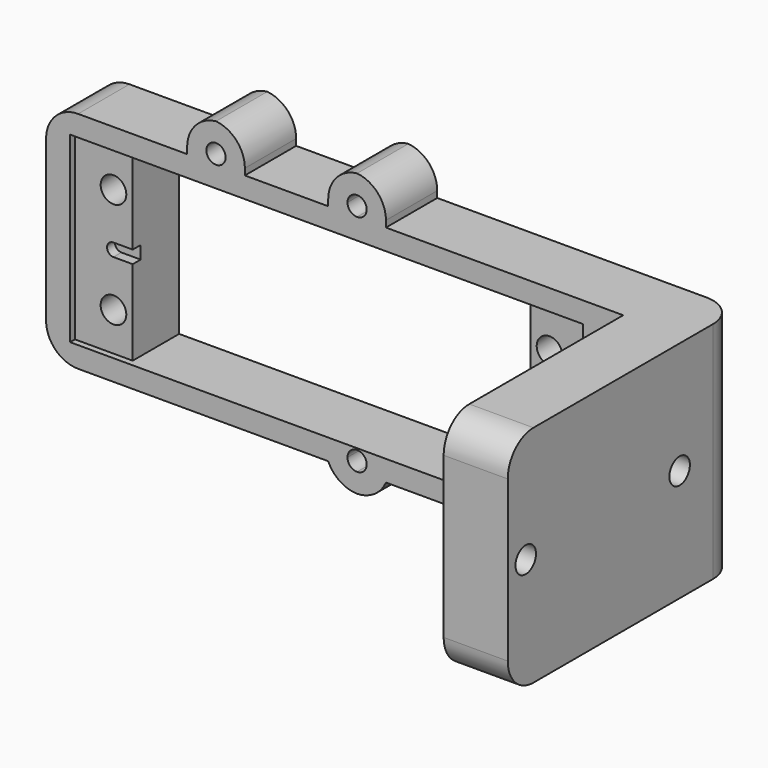
from build123d import *

# Parameters (mm, degrees)
F2_DEPTH     = 35
F4_DEPTH     = 10
F3_R         = 2
F5_DEPTH     = 0.95
F6_DEPTH     = 2.5
F7_DEPTH     = 6
F8_W         = 9
F8_H         = 9.25
F8_R         = 1.5
F8_H_2       = 6.25
F9_DEPTH     = 10
F10_DEPTH    = 10
F11_R        = 2
F12_DEPTH    = 6
F13_T1_DEPTH = 35
F13_T3_DEPTH = 35
F13_T5_DEPTH = 60
F13_T7_DEPTH = 32.9128784748


# Not quite as in the source:
# - a fillet or chamfer that OpenCascade refuses, or shapes differently, is made with other operations: its cross-section is extruded or revolved along the edge and cut away or added


with BuildPart() as f2:
    # F1 (on Top) → F2 (new body)
    with BuildSketch(Plane.XY):
        Polygon((50, -22.5), (50, 22.5), (-50, 22.5), (-50, 12.5), (40, 12.5), (40, -22.5), align=None)
    extrude(amount=F2_DEPTH)

    # F3 (on face) → F4 (cut, through all)
    with BuildSketch(Plane.XZ.offset(-12.5)):
        with BuildLine():
            Line((-37.25, 3.25), (24.75, 3.25))
            Line((24.75, 3.25), (24.75, 16.5))
            ThreePointArc((24.75, 16.5), (23.75, 17.5), (24.75, 18.5))
            Line((24.75, 18.5), (24.75, 31.75))
            Line((24.75, 31.75), (-37.25, 31.75))
            Line((-37.25, 31.75), (-37.25, 18.5))
            ThreePointArc((-37.25, 18.5), (-36.25, 17.5), (-37.25, 16.5))
            Line((-37.25, 16.5), (-37.25, 3.25))
        make_face()
        with BuildLine():
            Line((-37.25, 17.5), (-37.25, 16.5))
            ThreePointArc((-37.25, 16.5), (-36.25, 17.5), (-37.25, 18.5))
            Line((-37.25, 18.5), (-37.25, 17.5))
        make_face()
        with BuildLine():
            ThreePointArc((24.75, 18.5), (23.75, 17.5), (24.75, 16.5))
            Line((24.75, 16.5), (24.75, 17.5))
            Line((24.75, 17.5), (24.75, 18.5))
        make_face()
    extrude(amount=-F4_DEPTH, mode=Mode.SUBTRACT)

    # F3 (on face) → F5 (cut)
    with BuildSketch(Plane.XZ.offset(-12.5)):
        with BuildLine():
            Line((-43.25, 3.25), (-37.25, 3.25))
            Line((-37.25, 3.25), (-37.25, 16.5))
            Line((-37.25, 16.5), (-40.25, 16.5))
            ThreePointArc((-40.25, 16.5), (-41.25, 17.5), (-40.25, 18.5))
            Line((-40.25, 18.5), (-37.25, 18.5))
            Line((-37.25, 18.5), (-37.25, 31.75))
            Line((-37.25, 31.75), (-43.25, 31.75))
            Line((-43.25, 31.75), (-46.25, 31.75))
            Line((-46.25, 31.75), (-46.25, 3.25))
            Line((-46.25, 3.25), (-43.25, 3.25))
        make_face()
        with Locations((-40.25, 9.25)):
            Circle(F3_R, mode=Mode.SUBTRACT)
        with Locations((-40.25, 25.75)):
            Circle(F3_R, mode=Mode.SUBTRACT)
        with BuildLine():
            Line((27.75, 3.25), (30.75, 3.25))
            Line((30.75, 3.25), (33.75, 3.25))
            Line((33.75, 3.25), (33.75, 31.75))
            Line((33.75, 31.75), (30.75, 31.75))
            Line((30.75, 31.75), (24.75, 31.75))
            Line((24.75, 31.75), (24.75, 18.5))
            Line((24.75, 18.5), (27.75, 18.5))
            ThreePointArc((27.75, 18.5), (28.75, 17.5), (27.75, 16.5))
            Line((27.75, 16.5), (24.75, 16.5))
            Line((24.75, 16.5), (24.75, 3.25))
            Line((24.75, 3.25), (27.75, 3.25))
        make_face()
        with Locations((27.75, 9.25)):
            Circle(F3_R, mode=Mode.SUBTRACT)
        with Locations((27.75, 25.75)):
            Circle(F3_R, mode=Mode.SUBTRACT)
        with BuildLine():
            Line((-40.25, 16.5), (-37.25, 16.5))
            Line((-37.25, 16.5), (-37.25, 17.5))
            Line((-37.25, 17.5), (-37.25, 18.5))
            Line((-37.25, 18.5), (-40.25, 18.5))
            ThreePointArc((-40.25, 18.5), (-41.25, 17.5), (-40.25, 16.5))
        make_face()
        with BuildLine():
            Line((24.75, 17.5), (24.75, 16.5))
            Line((24.75, 16.5), (27.75, 16.5))
            ThreePointArc((27.75, 16.5), (28.75, 17.5), (27.75, 18.5))
            Line((27.75, 18.5), (24.75, 18.5))
            Line((24.75, 18.5), (24.75, 17.5))
        make_face()
    extrude(amount=-F5_DEPTH, mode=Mode.SUBTRACT)

    # F3 (on face) → F6 (cut)
    with BuildSketch(Plane.XZ.offset(-12.5)):
        with BuildLine():
            Line((-40.25, 16.5), (-37.25, 16.5))
            Line((-37.25, 16.5), (-37.25, 17.5))
            Line((-37.25, 17.5), (-37.25, 18.5))
            Line((-37.25, 18.5), (-40.25, 18.5))
            ThreePointArc((-40.25, 18.5), (-41.25, 17.5), (-40.25, 16.5))
        make_face()
        with BuildLine():
            Line((24.75, 17.5), (24.75, 16.5))
            Line((24.75, 16.5), (27.75, 16.5))
            ThreePointArc((27.75, 16.5), (28.75, 17.5), (27.75, 18.5))
            Line((27.75, 18.5), (24.75, 18.5))
            Line((24.75, 18.5), (24.75, 17.5))
        make_face()
    extrude(amount=-F6_DEPTH, mode=Mode.SUBTRACT)

    # F3 (on face) → F7 (cut)
    with BuildSketch(Plane.XZ.offset(-12.5)):
        with Locations((-40.25, 25.75)):
            Circle(F3_R)
        with Locations((-40.25, 9.25)):
            Circle(F3_R)
        with Locations((27.75, 9.25)):
            Circle(F3_R)
        with Locations((27.75, 25.75)):
            Circle(F3_R)
    extrude(amount=-F7_DEPTH, mode=Mode.SUBTRACT)

    # F8 (on face) → F9 (join, through all)
    with BuildSketch(Plane(origin=(0, 22.5, 0), x_dir=(-1, 0, 0), z_dir=(0, 1, 0))):
        with Locations((1.5, 36.375)):
            Rectangle(F8_W, F8_H)
        with Locations((1.5, 36.5)):
            Circle(F8_R, mode=Mode.SUBTRACT)
        with Locations((1.5, 0.125)):
            Rectangle(F8_W, F8_H_2)
        with Locations((1.5, 1.5)):
            Circle(F8_R, mode=Mode.SUBTRACT)
        with Locations((23.5, 36.375)):
            Rectangle(F8_W, F8_H)
        with Locations((23.5, 36.5)):
            Circle(F8_R, mode=Mode.SUBTRACT)
        with BuildLine():
            ThreePointArc((3, 36.5), (0.4393398187, 37.5606601622), (1.5000000271, 35))
            ThreePointArc((1.5000000271, 35), (2.5606601813, 35.4393398378), (3, 36.5))
        make_face()
    extrude(amount=-F9_DEPTH)

    # F8 (on face) → F10 (cut, through all)
    with BuildSketch(Plane(origin=(0, 22.5, 0), x_dir=(-1, 0, 0), z_dir=(0, 1, 0))):
        with BuildLine():
            ThreePointArc((3, 1.5), (0.4393398305, 2.560660174), (1.4999999936, 0))
            ThreePointArc((1.4999999936, 0), (2.5606601695, 0.439339826), (3, 1.5))
        make_face()
        with BuildLine():
            ThreePointArc((3, 36.5), (0.4393398187, 37.5606601622), (1.5000000271, 35))
            ThreePointArc((1.5000000271, 35), (2.5606601813, 35.4393398378), (3, 36.5))
        make_face()
    extrude(amount=-F10_DEPTH, mode=Mode.SUBTRACT)

    # F11 (on face) → F12 (cut)
    with BuildSketch(Plane.YZ.offset(50)):
        with Locations((-19, 17.5)):
            Circle(F11_R)
        with Locations((11, 17.5)):
            Circle(F11_R)
    extrude(amount=-F12_DEPTH, mode=Mode.SUBTRACT)

    # F13: fillet of radius 5 on 11 edges, made by hand

    # F13_s2 → F13_t1 (cut)
    with BuildSketch(Plane.XZ.offset(-35)):
        with BuildLine():
            ThreePointArc((-50, 30), (-48.5355339059, 33.5355339059), (-45, 35))
            Line((-45, 35), (-50, 35))
            Line((-50, 35), (-50, 30))
        make_face()
        with BuildLine():
            ThreePointArc((-45, 0), (-48.5355339059, 1.4644660941), (-50, 5))
            Line((-50, 5), (-50, 0))
            Line((-50, 0), (-45, 0))
        make_face()
        with BuildLine():
            ThreePointArc((-1, 41), (-4.5355339059, 39.5355339059), (-6, 36))
            Line((-6, 36), (-6, 41))
            Line((-6, 41), (-1, 41))
        make_face()
        with BuildLine():
            ThreePointArc((3, 36), (1.5355339059, 39.5355339059), (-2, 41))
            Line((-2, 41), (3, 41))
            Line((3, 41), (3, 36))
        make_face()
        with BuildLine():
            ThreePointArc((-28, 36), (-26.5355339059, 39.5355339059), (-23, 41))
            Line((-23, 41), (-28, 41))
            Line((-28, 41), (-28, 36))
        make_face()
        with BuildLine():
            ThreePointArc((-19, 36), (-20.4644660941, 39.5355339059), (-24, 41))
            Line((-24, 41), (-19, 41))
            Line((-19, 41), (-19, 36))
        make_face()
    extrude(amount=F13_T1_DEPTH, mode=Mode.SUBTRACT)

    # F13_s4 → F13_t3 (cut)
    with BuildSketch(Plane.YZ.offset(27.5)):
        with BuildLine():
            ThreePointArc((-22.5, 30), (-21.0355339059, 33.5355339059), (-17.5, 35))
            Line((-17.5, 35), (-22.5, 35))
            Line((-22.5, 35), (-22.5, 30))
        make_face()
        with BuildLine():
            ThreePointArc((-22.5, 5), (-21.0355339059, 1.4644660941), (-17.5, 0))
            Line((-17.5, 0), (-22.5, 0))
            Line((-22.5, 0), (-22.5, 5))
        make_face()
    extrude(amount=F13_T3_DEPTH, mode=Mode.SUBTRACT)

    # F13_s6 → F13_t5 (cut)
    with BuildSketch(Plane.XY.offset(-12.5)):
        with BuildLine():
            ThreePointArc((50, 17.5), (48.5355339059, 21.0355339059), (45, 22.5))
            Line((45, 22.5), (50, 22.5))
            Line((50, 22.5), (50, 17.5))
        make_face()
    extrude(amount=F13_T5_DEPTH, mode=Mode.SUBTRACT)

    # F13_s8 → F13_t7 (cut)
    with BuildSketch(Plane.XZ.offset(-33.9564392374)):
        with BuildLine():
            ThreePointArc((3, 0), (1.1560370926, -2.1833001327), (-1.582575695, -3))
            Line((-1.582575695, -3), (3, -3))
            Line((3, -3), (3, 0))
        make_face()
        with BuildLine():
            ThreePointArc((-1.417424305, -3), (-4.1560370926, -2.1833001327), (-6, 0))
            Line((-6, 0), (-6, -3))
            Line((-6, -3), (-1.417424305, -3))
        make_face()
    extrude(amount=F13_T7_DEPTH, mode=Mode.SUBTRACT)


solid = f2.part
